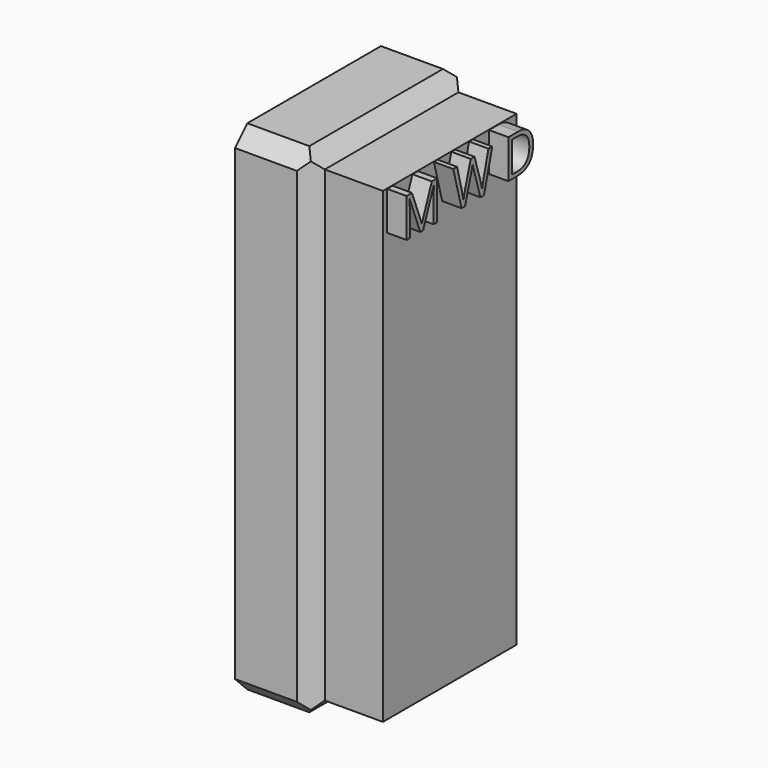
from build123d import *

# Parameters (mm, degrees)
F0_W          = 39.5231544971
F0_H          = 60.2282211185
F1_DEPTH      = 25.4
F2_DEPTH      = 103.17132622
F3_DEPTH      = 25.4
F4_SIZE       = 5.08
F5_SIZE       = 5.08
F6_SIZE       = 5.08
F7_SIZE       = 5.08
F8_SIZE       = 5.08
F9_SIZE       = 5.08
F10_SIZE      = 5.08
F11_SIZE      = 5.08
F12_TEXT_SIZE = 17.7739332006
F13_DEPTH     = 25.4
F14_DEPTH     = 19.05


# Not quite as in the source:
# - Text() gives the source's letters only with a copy of the font that has no kerning and outlines rounded to 1/6400 em; it was checked with that copy


with BuildPart() as f1:
    # F0 (on Right) → F1 (new body)
    with BuildSketch(Plane.YZ):
        with Locations((19.7615772486, 30.1141105592)):
            Rectangle(F0_W, F0_H)
    extrude(amount=F1_DEPTH)

    # F2 (add): a face of the model
    f2_faces = [f1.faces().sort_by_distance(p)[0] for p in [
        (12.7, 19.7615772486, 0),
    ]]
    extrude(f2_faces, amount=F2_DEPTH)

    # F3 (add): a face of the model
    f3_faces = [f1.faces().sort_by_distance(p)[0] for p in [
        (12.7, 39.5231544971, -21.4715525508),
    ]]
    extrude(f3_faces, amount=F3_DEPTH)

    # F4
    f4_edges = [f1.edges().sort_by_distance(p)[0] for p in [
        (12.7, 64.923154, -103.171326),
    ]]
    chamfer(f4_edges, length=F4_SIZE)

    # F5
    f5_edges = [f1.edges().sort_by_distance(p)[0] for p in [
        (25.4, 64.923154, -18.931553),
    ]]
    chamfer(f5_edges, length=F5_SIZE)

    # F6
    f6_edges = [f1.edges().sort_by_distance(p)[0] for p in [
        (10.16, 64.923154, 60.228221),
    ]]
    chamfer(f6_edges, length=F6_SIZE)

    # F7
    f7_edges = [f1.edges().sort_by_distance(p)[0] for p in [
        (25.4, 29.921577, -103.171326),
    ]]
    chamfer(f7_edges, length=F7_SIZE)

    # F8
    f8_edges = [f1.edges().sort_by_distance(p)[0] for p in [
        (25.4, 29.921577, 60.228221),
    ]]
    chamfer(f8_edges, length=F8_SIZE)

    # F9
    f9_edges = [f1.edges().sort_by_distance(p)[0] for p in [
        (25.4, 0, -21.471553),
    ]]
    chamfer(f9_edges, length=F9_SIZE)

    # F10
    f10_edges = [f1.edges().sort_by_distance(p)[0] for p in [
        (10.16, 0, -103.171326),
    ]]
    chamfer(f10_edges, length=F10_SIZE)

    # F11
    f11_edges = [f1.edges().sort_by_distance(p)[0] for p in [
        (10.16, 0, 60.228221),
    ]]
    chamfer(f11_edges, length=F11_SIZE)

    # F12 (on face) → F13 (join)
    with BuildSketch(Plane.YZ.offset(25.4)):
        with Locations((5.08, 42.3509892141)):
            Text('M W D', F12_TEXT_SIZE, font='Open Sans', text_align=(TextAlign.LEFT, TextAlign.BOTTOM))
    extrude(amount=F13_DEPTH)

    # F14 (add): a face of the model
    f14_faces = [f1.faces().sort_by_distance(p)[0] for p in [
        (25.4, 32.3227077115, -23.6420320932),
    ]]
    extrude(f14_faces, amount=F14_DEPTH)


solid = f1.part
